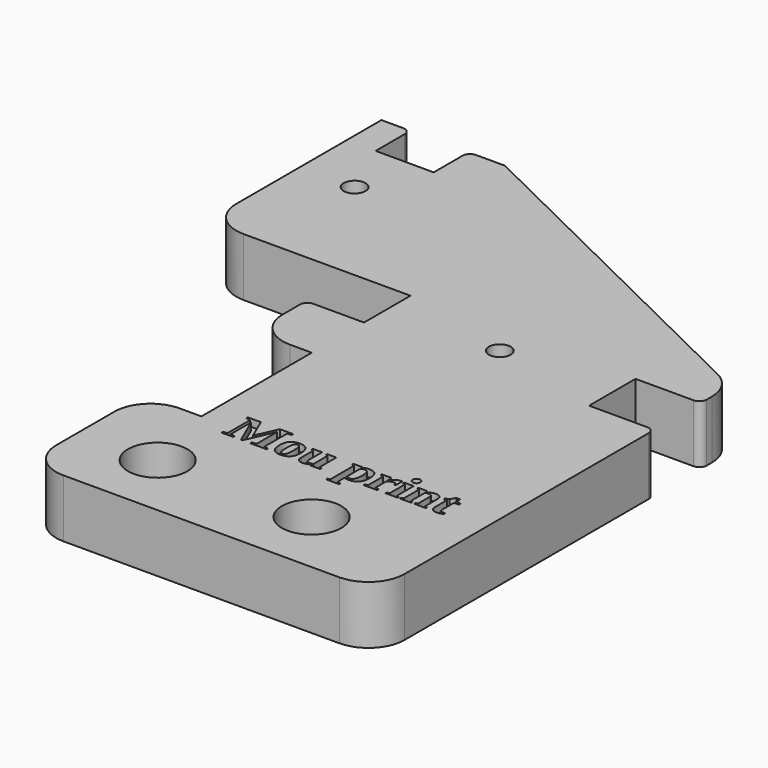
from build123d import *

# Parameters (mm, degrees)
F0_R         = 4.1
F0_R_2       = 1.5
F1_DEPTH     = 8
F2_R         = 1
F3_TEXT_SIZE = 6.9444444444
F4_DEPTH     = 1


# Not quite as in the source:
# - Text() gives the source's letters only with a copy of the font that has no kerning and outlines rounded to 1/6400 em; it was checked with that copy


with BuildPart() as f1:
    # F0 (on Top) → F1 (new body)
    with BuildSketch(Plane.XY):
        with BuildLine():
            ThreePointArc((-32.5311045349, -35.0281436741), (-31.0666384408, -38.5636775801), (-27.5311045349, -40.0281436741))
            Line((-27.5311045349, -40.0281436741), (10.4688954651, -40.0281436741))
            ThreePointArc((10.4688954651, -40.0281436741), (14.0044293711, -38.5636775801), (15.4688954651, -35.0281436741))
            Line((15.4688954651, -35.0281436741), (15.4688954651, 7.9718563259))
            Line((15.4688954651, 7.9718563259), (6.4688954651, 7.9718563259))
            Line((6.4688954651, 7.9718563259), (6.4688954651, 15.9718563259))
            Line((6.4688954651, 15.9718563259), (15.4688954651, 15.9718563259))
            Line((15.4688954651, 15.9718563259), (15.4688954651, 17.854416396))
            ThreePointArc((15.4688954651, 17.854416396), (14.7117677485, 20.4997962907), (12.6696815503, 22.3440200096))
            Line((12.6696815503, 22.3440200096), (-35.5311045349, 45.9718563259))
            Line((-35.5311045349, 45.9718563259), (-40.5311045349, 45.9718563259))
            Line((-40.5311045349, 45.9718563259), (-40.5311045349, 39.9718563259))
            Line((-40.5311045349, 39.9718563259), (-48.5311045349, 39.9718563259))
            Line((-48.5311045349, 39.9718563259), (-48.5311045349, 45.9718563259))
            Line((-48.5311045349, 45.9718563259), (-52.5311045349, 45.9718563259))
            Line((-52.5311045349, 45.9718563259), (-52.5311045349, 20.9718563259))
            ThreePointArc((-52.5311045349, 20.9718563259), (-51.0666384408, 17.4363224199), (-47.5311045349, 15.9718563259))
            Line((-47.5311045349, 15.9718563259), (-24.5311045349, 15.9718563259))
            Line((-24.5311045349, 15.9718563259), (-24.5311045349, 7.9718563259))
            Line((-24.5311045349, 7.9718563259), (-32.5311045349, 7.9718563259))
            Line((-32.5311045349, 7.9718563259), (-32.5311045349, 3.9718563259))
            ThreePointArc((-32.5311045349, 3.9718563259), (-31.0666384408, 0.4363224199), (-27.5311045349, -1.0281436741))
            Line((-27.5311045349, -1.0281436741), (-24.5311045349, -1.0281436741))
            Line((-24.5311045349, -1.0281436741), (-24.5311045349, -20.0281436741))
            Line((-24.5311045349, -20.0281436741), (-27.5311045349, -20.0281436741))
            ThreePointArc((-27.5311045349, -20.0281436741), (-31.0666384408, -21.4926097682), (-32.5311045349, -25.0281436741))
            Line((-32.5311045349, -25.0281436741), (-32.5311045349, -35.0281436741))
        make_face()
        with Locations((-21.8311045349, -30.9281436741)):
            Circle(F0_R, mode=Mode.SUBTRACT)
        with Locations((-0.6311045349, -30.9281436741)):
            Circle(F0_R, mode=Mode.SUBTRACT)
        with Locations((-45.0311045349, 31.9718563259)):
            Circle(F0_R_2, mode=Mode.SUBTRACT)
        with Locations((-9.0311045349, 11.9718563259)):
            Circle(F0_R_2, mode=Mode.SUBTRACT)
    extrude(amount=F1_DEPTH)

    # F2
    f2_edges = [f1.edges().sort_by_distance(p)[0] for p in [
        (-48.531105, 45.971856, 4),
        (-40.531105, 45.971856, 4),
        (15.468895, 15.971856, 4),
        (15.468895, 7.971856, 4),
        (-32.531105, 7.971856, 4),
    ]]
    fillet(f2_edges, radius=F2_R)

    # F3 (on face) → F4 (cut)
    with BuildSketch(Plane.XY.offset(8)):
        with Locations((-20.6074933418, -21.6281414032)):
            Text('Mou print', F3_TEXT_SIZE, font='Tinos', font_style=FontStyle.BOLD, text_align=(TextAlign.LEFT, TextAlign.BOTTOM))
    extrude(amount=-F4_DEPTH, mode=Mode.SUBTRACT)


solid = f1.part
